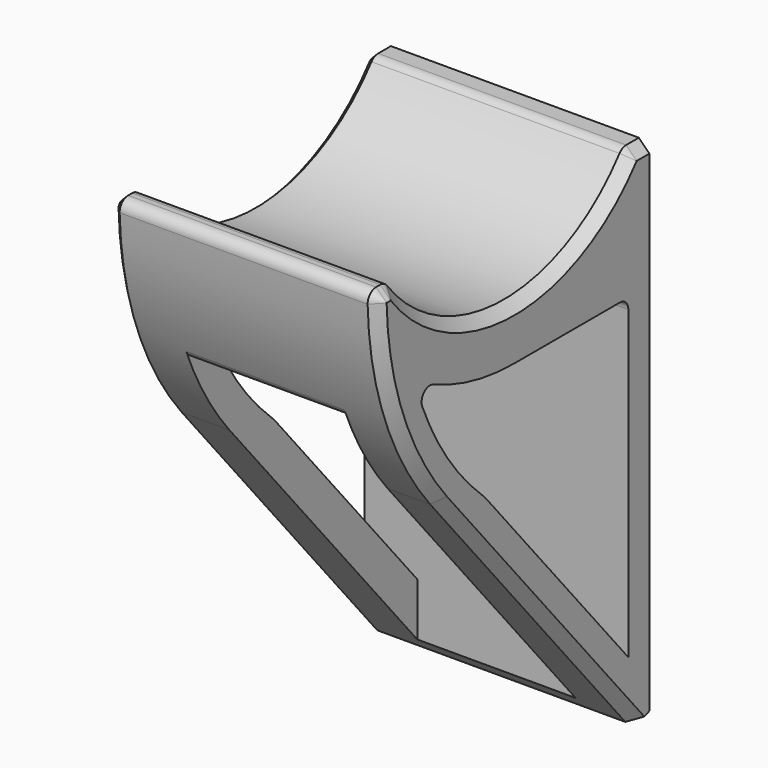
from build123d import *

# Parameters (mm, degrees)
F1_DEPTH       = 50
F4_DEPTH       = 25
F5_W           = 30
F5_H           = 60
F6_DEPTH       = 75
F8_D           = 4.4
F8_CSINK_D     = 8.96
F8_CSINK_ANGLE = 90
F9_R           = 2
F10_T1_DEPTH   = 30
F11_R          = 10
F12_SIZE       = 1.99999
F13_SIZE       = 1
F14_SIZE       = 5


# Not quite as in the source:
# - a fillet or chamfer that OpenCascade refuses, or shapes differently, is made with other operations: its cross-section is extruded or revolved along the edge and cut away or added
# - a fillet or chamfer is up to 0.001 mm smaller than in the source, because OpenCascade refuses the exact size


with BuildPart() as f1:
    # F0 (on Right) → F1 (new body)
    with BuildSketch(Plane.YZ):
        with BuildLine():
            Line((-49.4901207083, 58.9800291521), (0, 0))
            Line((0, 0), (0, 100))
            Line((0, 100), (-4, 100))
            ThreePointArc((-4, 100), (-32.2344149115, 86.0007850138), (-60.2787795686, 100.3769394581))
            Line((-60.2787795686, 100.3769394581), (-64.2787644391, 100.3879410703))
            ThreePointArc((-64.2787644391, 100.3879410703), (-60.5350609092, 78.3801837008), (-49.4901207083, 58.9800291521))
        make_face()
    extrude(amount=F1_DEPTH)

    # F3 (on offset) → F4 (cut, symmetric)
    with BuildSketch(Plane.YZ.offset(25)):
        with BuildLine():
            ThreePointArc((-32, 76), (-44.2642678148, 77.703490499), (-55.5999994652, 82.684989557))
            ThreePointArc((-55.5999994652, 82.684989557), (-49.1013266214, 68.5324924594), (-39.0785260857, 56.6132058929))
            Line((-39.0785260857, 56.6132058929), (-5, 16))
            Line((-5, 16), (-5, 76))
            Line((-5, 76), (-32, 76))
        make_face()
    extrude(amount=F4_DEPTH, both=True, mode=Mode.SUBTRACT)

    # F5 (on Top) → F6 (cut)
    with BuildSketch(Plane.XY):
        with Locations((25, -35)):
            Rectangle(F5_W, F5_H)
    extrude(amount=F6_DEPTH, mode=Mode.SUBTRACT)

    # F8 (through all)
    with Locations(Plane.XZ.offset(5)):
        with Locations((25.014353916, 63.602976501), (25.0169411302, 23.9024478942)):
            CounterSinkHole(F8_D / 2, F8_CSINK_D / 2, counter_sink_angle=F8_CSINK_ANGLE)

    # F9
    f9_edges = [f1.edges().sort_by_distance(p)[0] for p in [
        (25, -64.278764, 100.387941),
        (25, -60.27878, 100.376939),
        (25, -4, 100),
        (25, -59.21917, 75),
        (25, -55.599999, 82.68499),
        (25, -5, 76),
    ]]
    fillet(f9_edges, radius=F9_R)

    # F10: fillet of radius 2 on 1 edges, made by hand

    # F10_s2 → F10_t1 (cut)
    with BuildSketch(Plane.YZ.offset(10)):
        with BuildLine():
            ThreePointArc((-53.8387023607, 77.7281856581), (-54.0497056605, 75.8722525363), (-55.7014276886, 75))
            Line((-55.7014276886, 75), (-55.7014276886, 74.8))
            Line((-55.7014276886, 74.8), (-52.6458541761, 74.8))
            Line((-52.6458541761, 74.8), (-52.4647225466, 75.0848017263))
            ThreePointArc((-52.4647225466, 75.0848017263), (-53.6427658792, 77.7768016426), (-53.6524298279, 77.8010042239))
            Line((-53.6524298279, 77.8010042239), (-53.8387023607, 77.7281856581))
        make_face()
    extrude(amount=F10_T1_DEPTH, mode=Mode.SUBTRACT)

    # F11
    f11_edges = [f1.edges().sort_by_distance(p)[0] for p in [
        (45, -39.078526, 56.613206),
        (5, -39.078526, 56.613206),
    ]]
    fillet(f11_edges, radius=F11_R)

    # F12 (size 2 in the source; OpenCascade refuses exactly that, so slightly less here)
    f12_edges = [f1.edges().sort_by_distance(p)[0] for p in [
        (50, -32.228082, 86.000743),
        (50, -60.18128, 77.414084),
        (50, -63.689465, 99.780073),
        (50, -61.763987, 100.381024),
        (50, -60.395948, 100.173665),
        (50, -3.887164, 99.800901),
        (50, -1.508623, 100),
        (50, -24.74506, 29.490015),
    ]]
    chamfer(f12_edges, length=F12_SIZE)

    # F13
    f13_edges = [f1.edges().sort_by_distance(p)[0] for p in [
        (0, -1.508623, 100),
        (0, -3.887164, 99.800901),
        (0, -32.228082, 86.000743),
        (0, -60.395948, 100.173665),
        (0, -61.763987, 100.381024),
        (0, -63.689465, 99.780073),
        (0, -60.18128, 77.414084),
        (0, -24.74506, 29.490015),
    ]]
    chamfer(f13_edges, length=F13_SIZE)

    # F14
    f14_edges = [f1.edges().sort_by_distance(p)[0] for p in [
        (24.500005, 0, 0),
    ]]
    chamfer(f14_edges, length=F14_SIZE)


solid = f1.part
